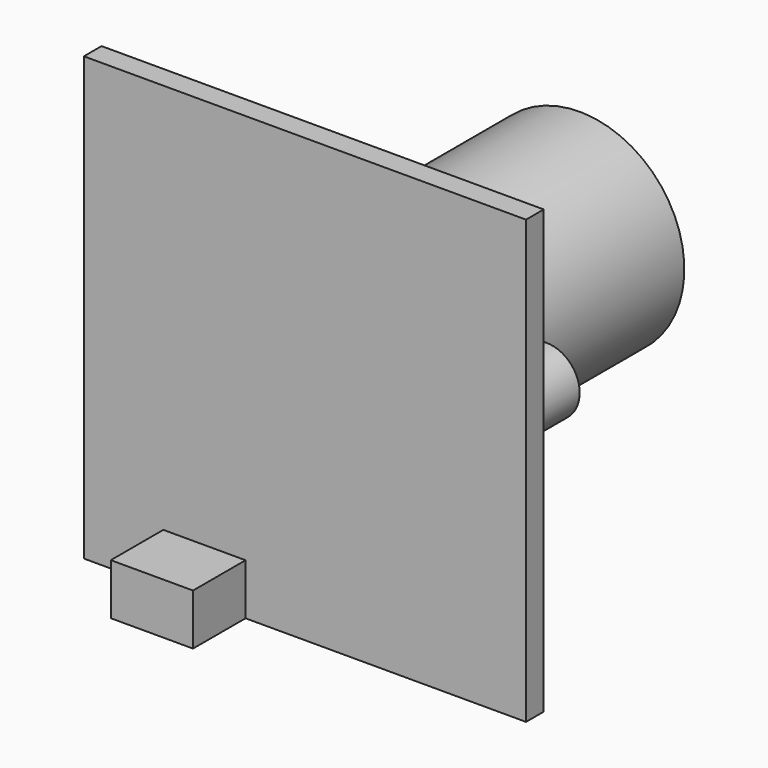
from build123d import *

# Parameters (mm, degrees)
F0_W     = 32
F0_H     = 32
F1_DEPTH = 1.6
F2_W     = 5.95
F2_H     = 3.7
F3_DEPTH = 4.75
F4_W     = 16.95
F4_H     = 16.95
F5_DEPTH = 7.75
F6_R     = 7.575
F7_DEPTH = 15.5
F8_R     = 1
F9_DEPTH = 7.75


# Not quite as in the source:
# - a pattern or mirror of a feature is missing from the dataset's text; its kind, count and spacing are read off the source's solid


with BuildPart() as f1:
    # F0 (on Front) → F1 (new body)
    with BuildSketch(Plane.XZ):
        Rectangle(F0_W, F0_H)
    extrude(amount=F1_DEPTH)

    # F2 (on face) → F3 (join)
    with BuildSketch(Plane.XZ.offset(1.6)):
        with Locations((-7.275, -14.15)):
            Rectangle(F2_W, F2_H)
    extrude(amount=F3_DEPTH)

    # F4 (on face) → F5 (join)
    with BuildSketch(Plane(origin=(0, 0, 0), x_dir=(-1, 0, 0), z_dir=(0, 1, 0))):
        Rectangle(F4_W, F4_H)
    extrude(amount=F5_DEPTH)

    # F6 (on face) → F7 (join)
    with BuildSketch(Plane(origin=(0, 7.75, 0), x_dir=(-1, 0, 0), z_dir=(0, 1, 0))):
        Circle(F6_R)
    extrude(amount=F7_DEPTH)

    # F8 (on face) → F9 (join)
    with BuildSketch(Plane(origin=(0, 0, 0), x_dir=(-1, 0, 0), z_dir=(0, 1, 0))):
        with BuildLine():
            Line((-8.475, 2.4), (-10, 2.4))
            ThreePointArc((-10, 2.4), (-12.4, 0), (-10, -2.4))
            Line((-10, -2.4), (-8.475, -2.4))
            Line((-8.475, -2.4), (-8.475, 2.4))
        make_face()
        with Locations((-10, 0)):
            Circle(F8_R, mode=Mode.SUBTRACT)
    f9 = extrude(amount=F9_DEPTH)

    # F9_copies: F9 across plane
    add(f9.mirror(Plane(origin=(0, 0, 0), x_dir=(0, 0, -1), z_dir=(-1, 0, 0))))


solid = f1.part
